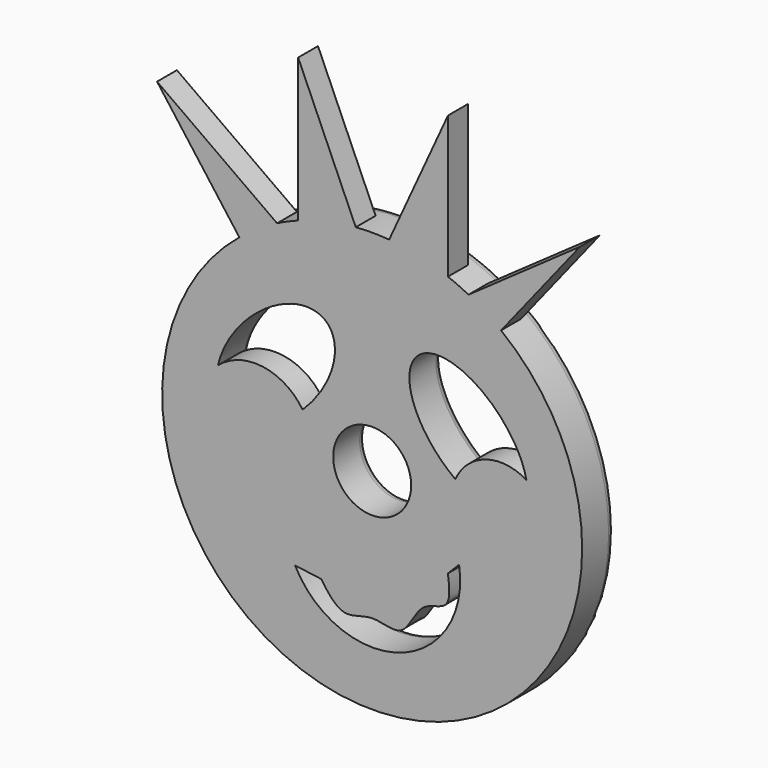
from build123d import *

# Parameters (mm, degrees)
F0_R     = 25.4
F1_DEPTH = 5
F2_R     = 4.7157463605
F3_DEPTH = 5
F4_R     = 5.9858344823
F4_R_2   = 6.8771684103
F5_DEPTH = 3
F6_R     = 1


# Not quite as in the source:
# - a feature names something its author has since deleted; it is built from what else it names


with BuildPart() as f1:
    # F0 (on Front) → F1 (new body)
    with BuildSketch(Plane.XZ):
        Circle(F0_R)
    extrude(amount=-F1_DEPTH)

    # F2 (on face) → F3 (cut)
    with BuildSketch(Plane.XZ):
        with BuildLine():
            add(Edge.make_bspline(
                [(5.4787751287, 14.0393581241), (-0.7613644186, 8.0220805736), (11.6041345431, 1.4428670645), (23.9696335047, -5.1363464445), (17.8442740904, 7.4601446151), (11.7189146761, 20.0566356747), (5.4787751287, 14.0393581241)],
                knots=[0, 0, 0, 2.0943951024, 2.0943951024, 4.1887902048, 4.1887902048, 6.2831853072, 6.2831853072, 6.2831853072], degree=2, weights=[1, 0.5, 1, 0.5, 1, 0.5, 1]))
        make_face()
        with BuildLine():
            add(Edge.make_bspline(
                [(-5.4787751287, 14.0393581241), (-11.7189146761, 20.0566356747), (-17.8442740904, 7.4601446151), (-23.9696335047, -5.1363464445), (-11.6041345431, 1.4428670645), (0.7613644186, 8.0220805736), (-5.4787751287, 14.0393581241)],
                knots=[0, 0, 0, 2.0943951024, 2.0943951024, 4.1887902048, 4.1887902048, 6.2831853072, 6.2831853072, 6.2831853072], degree=2, weights=[1, 0.5, 1, 0.5, 1, 0.5, 1]))
        make_face()
        with BuildLine():
            add(Edge.make_bspline(
                [(-9.3268435448, -13.0783319473), (-5.3570947234, -13.6419163621), (2.4941538192, -14.7565564853), (7.8622633612, -9.2576925536), (10.5161489919, -6.5391645767)],
                knots=[0, 0, 0, 0, 0.5056200679, 1, 1, 1, 1], degree=3))
            ThreePointArc((-9.3268435448, -13.0783319473), (3.3732506378, -18.2403565311), (10.5161489919, -6.5391645767))
        make_face()
        Circle(F2_R)
    extrude(amount=-F3_DEPTH, mode=Mode.SUBTRACT)

    # F4 (on Front) → F5 (join)
    with BuildSketch(Plane.XZ):
        Polygon((6.3790107723, 19.2006488251), (14.1368918121, 18.2225890458), (25.1383651048, 32.0631526411), (9.1684851795, 20.8250880241), (9.1684851795, 40.8442690969), (0, 20.8250880241), (-8.9521687478, 41.1240197718), (-8.9521687478, 20.8250880241), (-26.0172411799, 33.0111198127), (-13.7080065906, 16.5055599064), (-6.5881432822, 19.6455388269), (0.2679300325, 16.5055599064), align=None)
        with BuildLine():
            add(Edge.make_bspline(
                [(8.9071877301, -6.488062907), (9.2703313456, -8.4935320624), (9.9183873881, -12.0724367943), (5.6068314116, -11.6988309368), (4.0025303305, -17.0425236956), (-0.0779493441, -14.9823882563), (-3.872275032, -17.3296154794), (-6.088223658, -13.6780769927), (-7.3463311419, -11.6049116477)],
                knots=[0, 0, 0, 0, 0.180490001, 0.3220974589, 0.4922078924, 0.6459136955, 0.798967077, 1, 1, 1, 1], degree=3))
            Line((8.9071877301, -6.488062907), (0, -11.6049116477))
            Line((0, -11.6049116477), (-7.3463311419, -11.6049116477))
        make_face()
        with Locations((15.5406650156, 0)):
            Circle(F4_R)
        with Locations((-14.1438068822, 0)):
            Circle(F4_R_2)
    extrude(amount=-F5_DEPTH)

    # F6
    f6_edges = [f1.edges().sort_by_distance(p)[0] for p in [
        (-25.4, 5, 0),
        (1.711486, 5, -13.155),
        (3.373251, 5, -18.240357),
        (-4.715746, 5, 0),
        (-17.806014, 5, 1.255555),
        (17.806014, 5, 1.255555),
    ]]
    fillet(f6_edges, radius=F6_R)


solid = f1.part
